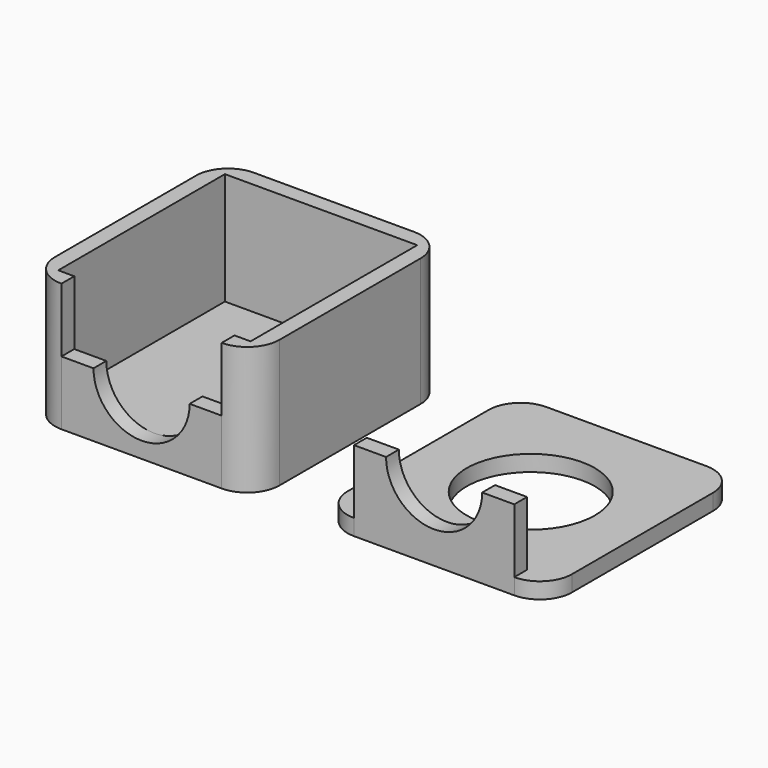
from build123d import *

# Parameters (mm, degrees)
F0_W      = 17.78
F0_H      = 19.05
F1_DEPTH  = 10.16
F2_W      = 15.24
F2_H      = 16.51
F3_DEPTH  = 8.89
F4_R      = 2.54
F5_W      = 2.54
F5_H      = 5.08
F6_DEPTH  = 1.27
F7_W      = 17.78
F7_H      = 19.05
F8_DEPTH  = 1.27
F9_R      = 2.54
F10_W     = 12.7
F10_H     = 1.27
F11_DEPTH = 5.08
F12_R     = 3.81
F13_DEPTH = 1.27
F14_R     = 5.08
F15_DEPTH = 1.27


# Not quite as in the source:
# - a feature names something its author has since deleted; it is built from what else it names


with BuildPart() as f1:
    # F0 (on Top) → F1 (new body)
    with BuildSketch(Plane.XY):
        with Locations((1.2571994369, -0.1732670812)):
            Rectangle(F0_W, F0_H)
    extrude(amount=F1_DEPTH)

    # F2 (on face) → F3 (cut)
    with BuildSketch(Plane.XY.offset(10.16)):
        with Locations((1.2571994369, -0.1732670812)):
            Rectangle(F2_W, F2_H)
    extrude(amount=-F3_DEPTH, mode=Mode.SUBTRACT)

    # F4
    f4_edges = [f1.edges().sort_by_distance(p)[0] for p in [
        (10.147199, 9.351733, 5.08),
        (-7.632801, 9.351733, 5.08),
        (-7.632801, -9.698267, 5.08),
        (10.147199, -9.698267, 5.08),
    ]]
    fillet(f4_edges, radius=F4_R)

    # F5 (on face) → F6 (cut)
    with BuildSketch(Plane.XZ.offset(9.6982670812)):
        with BuildLine():
            ThreePointArc((-2.5528005631, 5.08), (1.2571994369, 1.27), (5.0671994369, 5.08))
            ThreePointArc((5.0671994369, 5.08), (1.2571994369, 8.89), (-2.5528005631, 5.08))
        make_face()
        with Locations((-3.8228005631, 7.62)):
            Rectangle(F5_W, F5_H)
        with Locations((6.3371994369, 7.62)):
            Rectangle(F5_W, F5_H)
        with BuildLine():
            ThreePointArc((-2.5528005631, 5.08), (1.2571994369, 8.89), (5.0671994369, 5.08))
            Line((5.0671994369, 5.08), (5.0671994369, 10.16))
            Line((5.0671994369, 10.16), (-2.5528005631, 10.16))
            Line((-2.5528005631, 10.16), (-2.5528005631, 5.08))
        make_face()
    extrude(amount=-F6_DEPTH, mode=Mode.SUBTRACT)


with BuildPart() as f8:
    # F7 (on Top) → F8 (new body)
    with BuildSketch(Plane.XY):
        with Locations((24.3421698132, -0.0496563748)):
            Rectangle(F7_W, F7_H)
    extrude(amount=F8_DEPTH)

    # F9
    f9_edges = [f8.edges().sort_by_distance(p)[0] for p in [
        (15.45217, -9.574656, 0.635),
        (33.23217, -9.574656, 0.635),
        (33.23217, 9.475344, 0.635),
        (15.45217, 9.475344, 0.635),
    ]]
    fillet(f9_edges, radius=F9_R)

    # F10 (on face) → F11 (join)
    with BuildSketch(Plane.XY.offset(1.27)):
        with Locations((24.3421698132, -8.9396563748)):
            Rectangle(F10_W, F10_H)
    extrude(amount=F11_DEPTH)

    # F12 (on face) → F13 (cut)
    with BuildSketch(Plane.XZ.offset(9.5746563748)):
        with Locations((24.3421698132, 6.35)):
            Circle(F12_R)
    extrude(amount=-F13_DEPTH, mode=Mode.SUBTRACT)

    # F14 (on face) → F15 (cut)
    with BuildSketch(Plane.XY.offset(1.27)):
        with Locations((24.3421698132, 0)):
            Circle(F14_R)
    extrude(amount=-F15_DEPTH, mode=Mode.SUBTRACT)


solid = Compound([f1.part, f8.part])
